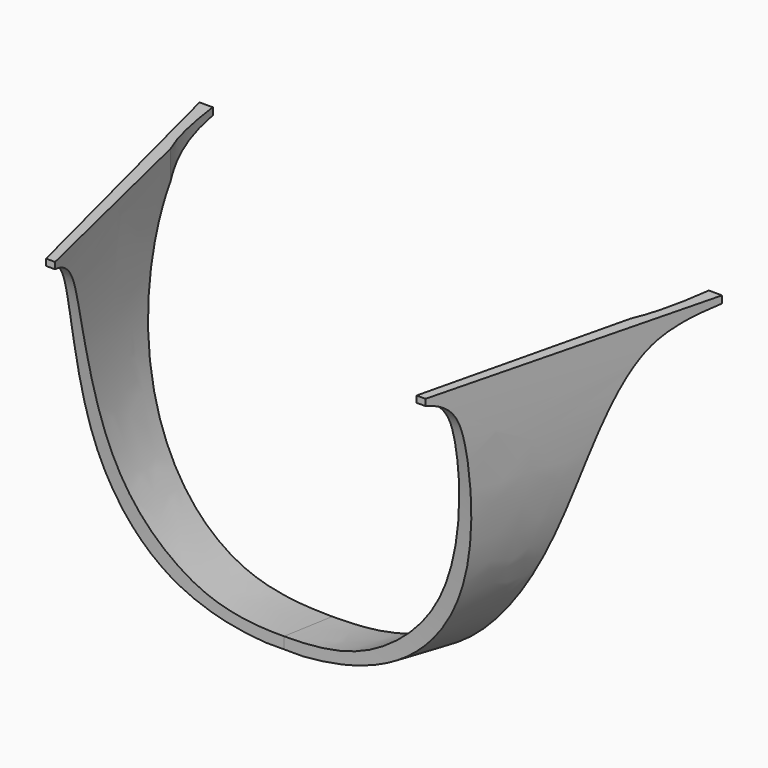
from build123d import *

# Parameters (mm, degrees)
F1_DEPTH      = 65
F3_DEPTH      = 40.0010001
F3_DEPTH_BACK = 85.9


# Not quite as in the source:
# - a feature names something its author has since deleted; it is built from what else it names


with BuildPart() as f1:
    # F0 (on Right) → F1 (new body, symmetric)
    with BuildSketch(Plane.YZ):
        with BuildLine():
            Line((35, 40), (-35, 40))
            Line((-35, 40), (-35, 38.3890762109))
            add(Edge.make_bspline(
                [(-35, 38.3890762109), (-28.3887613759, 36.7858445969), (-24.2082497767, 25.7315521456), (-20.8489437022, -8.7203708299), (-20, -24.070874226), (-20, -36.3589040935)],
                knots=[0.0448264701, 0.0448264701, 0.0448264701, 0.0448264701, 0.2770313204, 0.6498629592, 1, 1, 1, 1], degree=3))
            Line((-20, -36.3589040935), (-5, -40))
            add(Edge.make_bspline(
                [(35, 38.2211208172), (24.3591849947, 37.5670207986), (13.8787548205, 33.9950835571), (2.1031849423, 12.3507270988), (-4.1445688838, -17.3687620039), (-5, -30.6638973876), (-5, -40)],
                knots=[0.0630233334, 0.0630233334, 0.0630233334, 0.0630233334, 0.2726397053, 0.5030464591, 0.7661957364, 1, 1, 1, 1], degree=3))
            Line((35, 38.2211208172), (35, 40))
        make_face()
    extrude(amount=F1_DEPTH, both=True)

    # F2 (on Top) → F3 (cut, two sides)
    with BuildSketch(Plane.XY) as f3_sk:
        with BuildLine():
            add(Edge.make_bspline(
                [(0, -5), (-21.1868966551, -5), (-44.859775997, -1.3862829784), (-60.3499393631, 16.8039243987), (-62.8645139157, 46.5324734786), (-62.821932137, 46.3287681341), (-63.1294697523, 54.7901801765)],
                knots=[0, 0, 0, 0, 0.3413749666, 0.5765869346, 0.8280831413, 1, 1, 1, 1], degree=3))
            add(Edge.make_bspline(
                [(0, -5), (21.1868966551, -5), (44.859775997, -1.3862829784), (60.3499393631, 16.8039243987), (62.8645139157, 46.5324734786), (62.821932137, 46.3287681341), (63.1294697523, 54.7901801765)],
                knots=[0, 0, 0, 0, 0.3413749666, 0.5765869346, 0.8280831413, 1, 1, 1, 1], degree=3))
            Line((63.1294697523, 54.7901801765), (0, 54.7901801765))
            Line((0, 54.7901801765), (-63.1294697523, 54.7901801765))
        make_face()
    extrude(amount=-F3_DEPTH, mode=Mode.SUBTRACT)
    extrude(f3_sk.sketch, amount=F3_DEPTH_BACK, mode=Mode.SUBTRACT)

    # F7 (on plane+point) → F9 section 0
    with BuildSketch(Plane.XZ.offset(35)):
        with BuildLine():
            Line((45, 40.6529456377), (-45, 40.6529456377))
            add(Edge.make_bspline(
                [(-45, 40.6529456377), (-45, 21.3988348234), (-41.2938575358, -10.2833538762), (-24.5640150561, -26.074854919), (-12.3383639878, -31.8445574922), (0, -31.7242741585)],
                knots=[0, 0, 0, 0, 0.4293659783, 0.6961332157, 1, 1, 1, 1], degree=3))
            add(Edge.make_bspline(
                [(45, 40.6529456377), (45, 21.3988348234), (41.2938575358, -10.2833538762), (24.5640150561, -26.074854919), (12.3383639878, -31.8445574922), (0, -31.7242741585)],
                knots=[0, 0, 0, 0, 0.4293659783, 0.6961332157, 1, 1, 1, 1], degree=3))
        make_face()
    # F8 (on offset) → F9 section 1
    with BuildSketch(Plane(origin=(0, 35, 0), x_dir=(-1, 0, 0), z_dir=(0, 1, 0))):
        with BuildLine():
            Line((61.7376105536, 40.7376475632), (-61.7376105536, 40.7376475632))
            add(Edge.make_bspline(
                [(-61.7376105536, 40.7376475632), (-61.7376105536, 22.1820947396), (-61.6603638055, 3.8091101249), (-36.6777608388, -36.4594176552), (-16.6839537096, -40), (0, -40)],
                knots=[0, 0, 0, 0, 0.3375011143, 0.6744256061, 1, 1, 1, 1], degree=3))
            add(Edge.make_bspline(
                [(61.7376105536, 40.7376475632), (61.7376105536, 22.1820947396), (61.6603638055, 3.8091101249), (36.6777608388, -36.4594176552), (16.6839537096, -40), (0, -40)],
                knots=[0, 0, 0, 0, 0.3375011143, 0.6744256061, 1, 1, 1, 1], degree=3))
        make_face()
    loft(mode=Mode.SUBTRACT)

    # F7 (on plane+point) → F10 section 0
    with BuildSketch(Plane.XZ.offset(35)):
        with BuildLine():
            add(Edge.make_bspline(
                [(0, -34.911967814), (9.9495450076, -34.800420641), (26.2987176559, -30.2304553539), (44.9909741081, -10.8187434613), (47.4557727575, 18.3558147401), (47.2021177411, 45.2433638275)],
                knots=[0, 0, 0, 0, 0.2939421978, 0.5653395013, 1, 1, 1, 1], degree=3))
            add(Edge.make_bspline(
                [(0, -34.911967814), (-9.9495450076, -34.800420641), (-26.2987176559, -30.2304553539), (-44.9909741081, -10.8187434613), (-47.4557727575, 18.3558147401), (-47.2021177411, 45.2433638275)],
                knots=[0, 0, 0, 0, 0.2939421978, 0.5653395013, 1, 1, 1, 1], degree=3))
            Line((-47.2021177411, 45.2433638275), (-70.9189623594, 45.2433638275))
            Line((-70.9189623594, 45.2433638275), (-70.9189623594, -46.7069782317))
            Line((-70.9189623594, -46.7069782317), (0, -46.7069782317))
            Line((0, -46.7069782317), (70.9189623594, -46.7069782317))
            Line((70.9189623594, -46.7069782317), (70.9189623594, 45.2433638275))
            Line((70.9189623594, 45.2433638275), (47.2021177411, 45.2433638275))
        make_face()
    # F8 (on offset) → F10 section 1
    with BuildSketch(Plane(origin=(0, 35, 0), x_dir=(-1, 0, 0), z_dir=(0, 1, 0))):
        with BuildLine():
            add(Edge.make_bspline(
                [(-65, 53.6546695452), (-65, 28.6967538351), (-66.2320918701, 1.2821787191), (-39.930140464, -41.1659054757), (-14.0474298659, -42.2204924203), (0, -42.5526282684)],
                knots=[0, 0, 0, 0, 0.3711857647, 0.6921160123, 1, 1, 1, 1], degree=3))
            Line((-65, 53.6546695452), (-87.8087878227, 53.6546695452))
            Line((-87.8087878227, 53.6546695452), (-87.8087878227, -53.5140633583))
            Line((-87.8087878227, -53.5140633583), (0, -53.5140633583))
            Line((0, -53.5140633583), (87.8087878227, -53.5140633583))
            Line((87.8087878227, -53.5140633583), (87.8087878227, 53.6546695452))
            Line((87.8087878227, 53.6546695452), (65, 53.6546695452))
            add(Edge.make_bspline(
                [(65, 53.6546695452), (65, 28.6967538351), (66.2320918701, 1.2821787191), (39.930140464, -41.1659054757), (14.0474298659, -42.2204924203), (0, -42.5526282684)],
                knots=[0, 0, 0, 0, 0.3711857647, 0.6921160123, 1, 1, 1, 1], degree=3))
        make_face()
    loft(mode=Mode.SUBTRACT)


solid = f1.part
